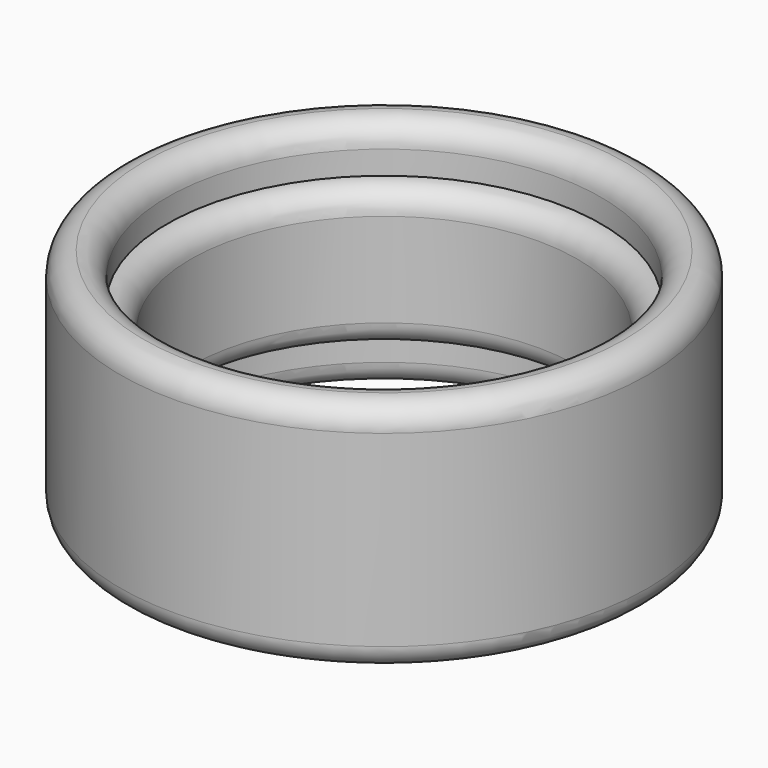
from build123d import *

# Parameters (mm, degrees)
F0_R     = 11.25
F0_R_2   = 9.25
F1_DEPTH = 10
F3_R     = 11.25
F3_R_2   = 8.25
F4_DEPTH = 6
F5_R     = 0.99999


# Not quite as in the source:
# - a fillet or chamfer is up to 0.001 mm smaller than in the source, because OpenCascade refuses the exact size


with BuildPart() as f1:
    # F0 (on Top) → F1 (new body)
    with BuildSketch(Plane.XY):
        Circle(F0_R)
        Circle(F0_R_2, mode=Mode.SUBTRACT)
    extrude(amount=F1_DEPTH)

    # F3 (on offset) → F4 (join)
    with BuildSketch(Plane.XY.offset(2)):
        Circle(F3_R)
        Circle(F3_R_2, mode=Mode.SUBTRACT)
    extrude(amount=F4_DEPTH)

    # F5 (radius 1 in the source; OpenCascade refuses exactly that, so slightly less here)
    f5_edges = [f1.edges().sort_by_distance(p)[0] for p in [
        (-8.25, 0, 2),
        (-8.25, 0, 8),
        (-9.25, 0, 10),
        (-11.25, 0, 10),
        (-11.25, 0, 0),
        (-9.25, 0, 0),
    ]]
    fillet(f5_edges, radius=F5_R)


solid = f1.part
